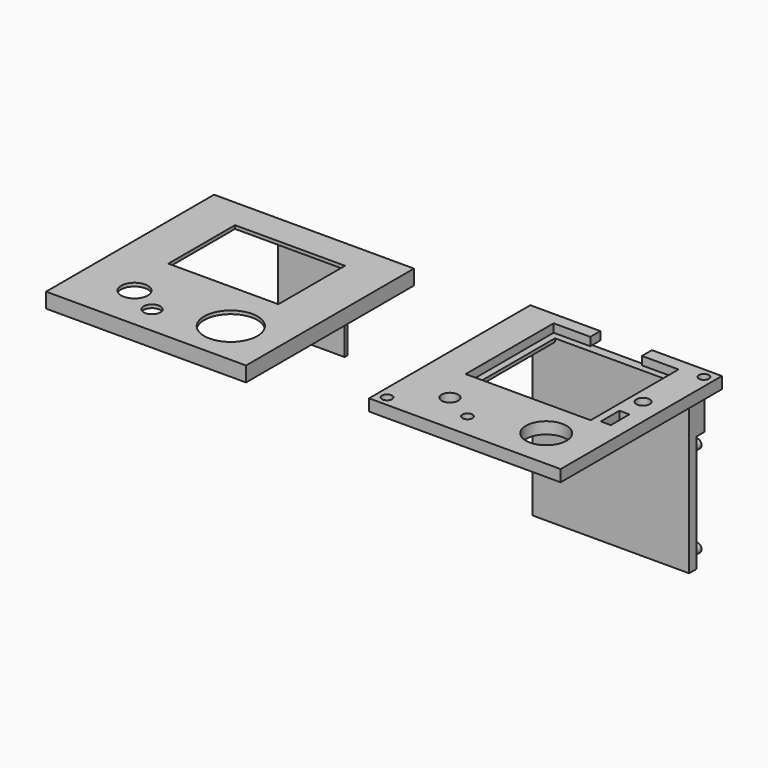
from build123d import *

# Parameters (mm, degrees)
F1_W      = 57.5
F1_H      = 60.5
F1_R      = 1.5
F1_R_2    = 2.5
F1_R_3    = 6.1
F1_W_2    = 3
F1_H_2    = 7
F1_W_3    = 37.5
F1_H_3    = 33
F1_R_4    = 2
F2_DEPTH  = 3.5
F4_W      = 37.5
F4_H      = 33
F4_W_2    = 33.5
F4_H_2    = 29
F5_DEPTH  = 1
F3_W      = 15.5
F3_H      = 3.75
F6_DEPTH  = 2.5
F8_DEPTH  = 5.75
F10_DEPTH = 3
F11_R     = 1.4
F12_DEPTH = 3
F0_W      = 58
F0_H      = 61
F0_R      = 4
F0_R_2    = 2.5
F0_R_3    = 8
F0_W_2    = 33
F0_H_2    = 25
F0_H_3    = 1
F13_DEPTH = 1
F14_DEPTH = 3.5
F15_W     = 20
F15_H     = 1
F16_DEPTH = 25


with BuildPart() as f2:
    # F1 (on Top) → F2 (new body)
    with BuildSketch(Plane.XY):
        with Locations((94.6610440163, 0)):
            Rectangle(F1_W, F1_H)
        with Locations((68.9110440163, -27.25)):
            Circle(F1_R, mode=Mode.SUBTRACT)
        with Locations((89.6610440163, -23)):
            Circle(F1_R, mode=Mode.SUBTRACT)
        with Locations((80.5110440163, -18.15)):
            Circle(F1_R_2, mode=Mode.SUBTRACT)
        with Locations((109.4110440163, -18.15)):
            Circle(F1_R_3, mode=Mode.SUBTRACT)
        with Locations((117.1610440163, -2)):
            Rectangle(F1_W_2, F1_H_2, mode=Mode.SUBTRACT)
        with Locations((94.6610440163, 10)):
            Rectangle(F1_W_3, F1_H_3, mode=Mode.SUBTRACT)
        with Locations((117.1610440163, 8.5)):
            Circle(F1_R_4, mode=Mode.SUBTRACT)
        with Locations((120.4110440163, 27.25)):
            Circle(F1_R, mode=Mode.SUBTRACT)
    extrude(amount=F2_DEPTH)

    # F4 (on face) → F5 (join)
    with BuildSketch(Plane(origin=(0, 0, 0), x_dir=(1, 0, 0), z_dir=(0, 0, -1))):
        with Locations((94.6610440163, -10)):
            Rectangle(F4_W, F4_H)
        with Locations((94.6610440163, -10)):
            Rectangle(F4_W_2, F4_H_2, mode=Mode.SUBTRACT)
    extrude(amount=-F5_DEPTH)

    # F3 (on face) → F6 (cut)
    with BuildSketch(Plane.XY.offset(3.5)):
        with Locations((94.6610440163, 28.375)):
            Rectangle(F3_W, F3_H)
    extrude(amount=-F6_DEPTH, mode=Mode.SUBTRACT)

    # F7 (on face) → F8 (join)
    with BuildSketch(Plane.XZ.offset(-24.5)):
        Polygon((77.9110440163, 0), (71.1610440163, 0), (71.1610440163, -48), (118.1610440163, -48), (118.1610440163, 0), (111.4110440163, 0), align=None)
    extrude(amount=-F8_DEPTH)

    # F9 (on face) → F10 (cut)
    with BuildSketch(Plane(origin=(0, 30.25, 0), x_dir=(-1, 0, 0), z_dir=(0, 1, 0))):
        Polygon((-105.1610440163, -13), (-118.1610440163, -13), (-118.1610440163, -48), (-71.1610440163, -48), (-71.1610440163, -13), (-84.1610440163, -13), (-86.9110440163, -13), align=None)
        Polygon((-105.1610440163, 1), (-105.1610440163, -13), (-86.9110440163, -13), (-84.1610440163, -13), (-84.1610440163, 1), (-86.9110440163, 1), (-102.4110440163, 1), align=None)
    extrude(amount=-F10_DEPTH, mode=Mode.SUBTRACT)

    # F11 (on face) → F12 (join)
    with BuildSketch(Plane(origin=(0, 27.25, 0), x_dir=(-1, 0, 0), z_dir=(0, 1, 0))):
        with Locations((-115.9110440163, -16.75)):
            Circle(F11_R)
        with Locations((-115.9110440163, -44.25)):
            Circle(F11_R)
        with Locations((-73.4110440163, -16.75)):
            Circle(F11_R)
        with Locations((-73.4110440163, -44.25)):
            Circle(F11_R)
    extrude(amount=F12_DEPTH)


with BuildPart() as f13:
    # F0 (on Top) → F13 (new body)
    with BuildSketch(Plane.XY):
        Rectangle(F0_W, F0_H)
        with Locations((-14.15, -18.15)):
            Circle(F0_R, mode=Mode.SUBTRACT)
        with Locations((-5, -23)):
            Circle(F0_R_2, mode=Mode.SUBTRACT)
        with Locations((14.75, -18.15)):
            Circle(F0_R_3, mode=Mode.SUBTRACT)
        with Locations((0, 10)):
            Rectangle(F0_W_2, F0_H_2, mode=Mode.SUBTRACT)
        Polygon((-29, -31.5), (-29, -30.5), (-29, 30.5), (-29, 31.5), (-30, 31.5), (-30, -31.5), align=None)
        with Locations((0, 31)):
            Rectangle(F0_W, F0_H_3)
        Polygon((29, 30.5), (29, -30.5), (29, -31.5), (30, -31.5), (30, 31.5), (29, 31.5), align=None)
        with Locations((0, -31)):
            Rectangle(F0_W, F0_H_3)
    extrude(amount=F13_DEPTH)

    # F0 (on Top) → F14 (join)
    with BuildSketch(Plane.XY):
        with Locations((0, 31)):
            Rectangle(F0_W, F0_H_3)
        Polygon((-29, -31.5), (-29, -30.5), (-29, 30.5), (-29, 31.5), (-30, 31.5), (-30, -31.5), align=None)
        with Locations((0, -31)):
            Rectangle(F0_W, F0_H_3)
        Polygon((29, 30.5), (29, -30.5), (29, -31.5), (30, -31.5), (30, 31.5), (29, 31.5), align=None)
    extrude(amount=-F14_DEPTH)

    # F15 (on face) → F16 (join)
    with BuildSketch(Plane(origin=(0, 0, -3.5), x_dir=(1, 0, 0), z_dir=(0, 0, -1))):
        with Locations((0, -31)):
            Rectangle(F15_W, F15_H)
    extrude(amount=F16_DEPTH)


solid = Compound([f2.part, f13.part])
